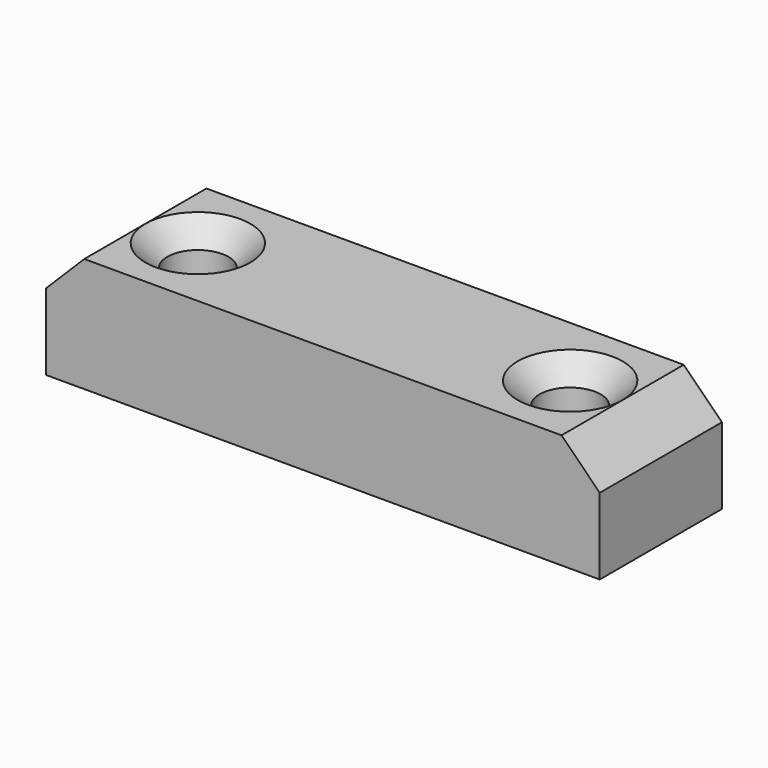
from build123d import *

# Parameters (mm, degrees)
F0_W           = 29
F0_H           = 6
F1_DEPTH       = 8
F2_R           = 5
F3_DEPTH       = 6
F5_D           = 3.2
F5_DEPTH       = 10
F5_CSINK_D     = 5.5
F5_CSINK_ANGLE = 90
F5_TIP         = 0.9613769904
F6_T1_DEPTH    = 18.2867319519


# Not quite as in the source:
# - a fillet or chamfer that OpenCascade refuses, or shapes differently, is made with other operations: its cross-section is extruded or revolved along the edge and cut away or added


with BuildPart() as f1:
    # F0 (on Front) → F1 (new body)
    with BuildSketch(Plane.XZ):
        with Locations((14.5, 3)):
            Rectangle(F0_W, F0_H)
    extrude(amount=F1_DEPTH)

    # F2 (on face) → F3 (cut)
    with BuildSketch(Plane(origin=(0, 0, 0), x_dir=(-1, 0, 0), z_dir=(0, 1, 0))):
        with Locations((-14.5, 0)):
            Circle(F2_R)
    extrude(amount=-F3_DEPTH, mode=Mode.SUBTRACT)

    # F5
    with Locations(Plane.XY.offset(6)):
        with Locations((4.75, -4), (24.25, -4)):
            CounterSinkHole(F5_D / 2, F5_CSINK_D / 2, depth=F5_DEPTH, counter_sink_angle=F5_CSINK_ANGLE)
            with Locations((0, 0, -(F5_DEPTH + F5_TIP / 2))):  # 118° drill point
                Cone(0, F5_D / 2, F5_TIP, mode=Mode.SUBTRACT)

    # F6: chamfer of 2 on 2 edges, made by hand

    # F6_s2 → F6_t1 (cut)
    with BuildSketch(Plane.XZ.offset(-5.1433659759)):
        Polygon((27, 6), (29, 4), (29, 6), align=None)
        Polygon((0, 4), (2, 6), (0, 6), align=None)
    extrude(amount=F6_T1_DEPTH, mode=Mode.SUBTRACT)


solid = f1.part
